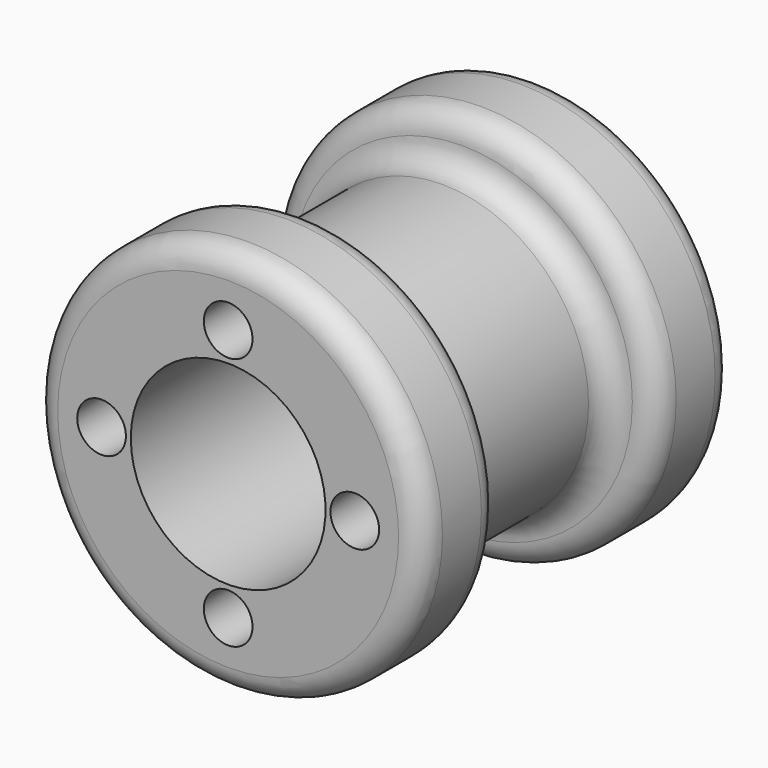
from build123d import *

# Parameters (mm, degrees)
F0_R     = 12.7
F1_DEPTH = 6.35
F2_R     = 9.525
F3_DEPTH = 12.7
F4_R     = 12.7
F5_DEPTH = 6.35
F7_D     = 12.7
F9_D     = 3.175
F9_DEPTH = 3.175
F9_TIP   = 0.9538662327
F10_R    = 1.58749


# Not quite as in the source:
# - a fillet or chamfer is up to 0.001 mm smaller than in the source, because OpenCascade refuses the exact size


with BuildPart() as f1:
    # F0 (on Front) → F1 (new body)
    with BuildSketch(Plane.XZ):
        Circle(F0_R)
    extrude(amount=F1_DEPTH)

    # F2 (on face) → F3 (join)
    with BuildSketch(Plane(origin=(0, 0, 0), x_dir=(-1, 0, 0), z_dir=(0, 1, 0))):
        Circle(F2_R)
    extrude(amount=F3_DEPTH)

    # F4 (on face) → F5 (join)
    with BuildSketch(Plane(origin=(0, 12.7, 0), x_dir=(-1, 0, 0), z_dir=(0, 1, 0))):
        Circle(F4_R)
    extrude(amount=F5_DEPTH)

    # F7 (through all)
    with Locations(Plane.XZ.offset(6.35)):
        with Locations((0, 0)):
            Hole(F7_D / 2)

    # F9
    with Locations(Plane.XZ.offset(6.35)):
        with Locations((0, 8.255), (-8.255, 0), (8.255, 0), (0, -8.255)):
            Hole(F9_D / 2, depth=F9_DEPTH)
            with Locations((0, 0, -(F9_DEPTH + F9_TIP / 2))):  # 118° drill point
                Cone(0, F9_D / 2, F9_TIP, mode=Mode.SUBTRACT)

    # F10 (radius 1.5875 in the source; OpenCascade refuses exactly that, so slightly less here)
    f10_edges = [f1.edges().sort_by_distance(p)[0] for p in [
        (12.7, 12.7, 0),
        (9.525, 12.7, 0),
        (-12.7, 0, 0),
        (9.525, 0, 0),
        (12.7, 19.05, 0),
        (-12.7, -6.35, 0),
    ]]
    fillet(f10_edges, radius=F10_R)


solid = f1.part
